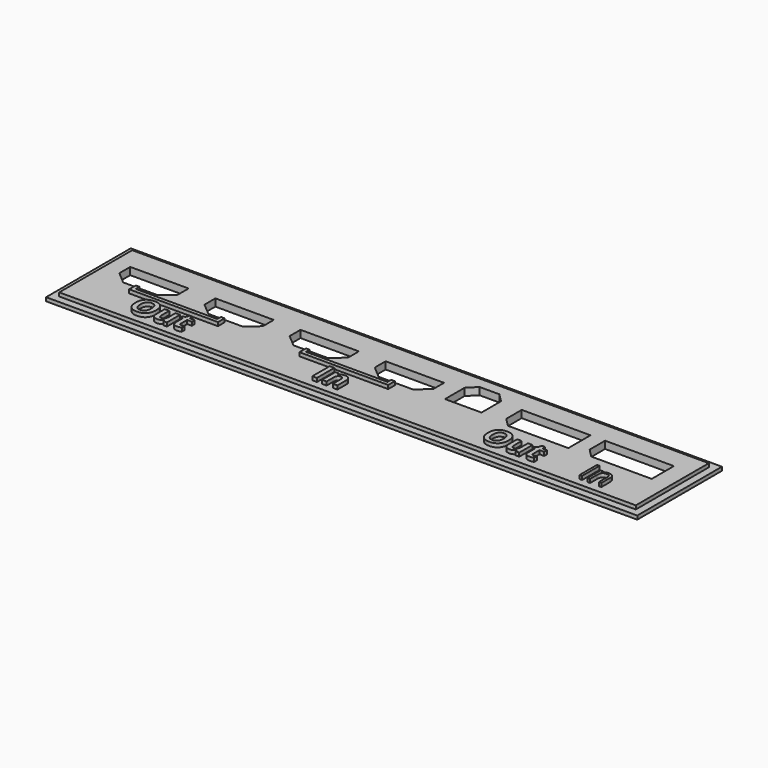
from build123d import *

# Parameters (mm, degrees)
F2_W          = 158
F2_H          = 25
F3_DEPTH      = 2
F2_W_2        = 162
F2_H_2        = 29
F4_DEPTH      = 1
F9_DEPTH      = 2
F10_OFFSET    = 0.5
F11_TEXT_SIZE = 8.3333333333
F12_DEPTH     = 1


# Not quite as in the source:
# - Text() gives the source's letters only with a copy of the font that has no kerning and outlines rounded to 1/6400 em; it was checked with that copy


with BuildPart() as f3:
    # F2 (on Top) → F3 (new body)
    with BuildSketch(Plane.XY):
        with Locations((-79, 12.5)):
            Rectangle(F2_W, F2_H)
    extrude(amount=F3_DEPTH)

    # F2 (on Top) → F4 (join)
    with BuildSketch(Plane.XY):
        with Locations((-79, 12.5)):
            Rectangle(F2_W_2, F2_H_2)
        with Locations((-79, 12.5)):
            Rectangle(F2_W, F2_H, mode=Mode.SUBTRACT)
    extrude(amount=F4_DEPTH)


with BuildPart() as f9:
    # F6 (on face) → F9 (new body, through all)
    with BuildSketch(Plane.XY.offset(2)):
        Polygon((-138, 18.2), (-145.5, 18.2), (-153, 18.2), (-153, 15.2), (-150, 12.65), (-145.5, 12.65), (-141, 12.65), (-138, 15.2), align=None)
    extrude(amount=-F9_DEPTH)


with BuildPart() as f9b:
    # F6 (on face) → F9, piece 2 (new body, through all)
    with BuildSketch(Plane.XY.offset(2)):
        Polygon((-114.67, 18.2), (-122.17, 18.2), (-129.67, 18.2), (-129.67, 15.2), (-126.67, 12.65), (-122.17, 12.65), (-117.67, 12.65), (-114.67, 15.2), align=None)
    extrude(amount=-F9_DEPTH)


with BuildPart() as f9c:
    # F6 (on face) → F9, piece 3 (new body, through all)
    with BuildSketch(Plane.XY.offset(2)):
        Polygon((-91.34, 18.2), (-98.84, 18.2), (-106.34, 18.2), (-106.34, 15.2), (-103.34, 12.65), (-98.84, 12.65), (-94.34, 12.65), (-91.34, 15.2), align=None)
    extrude(amount=-F9_DEPTH)


with BuildPart() as f9d:
    # F6 (on face) → F9, piece 4 (new body, through all)
    with BuildSketch(Plane.XY.offset(2)):
        Polygon((-68.01, 18.2), (-75.51, 18.2), (-83.01, 18.2), (-83.01, 15.2), (-80.01, 12.65), (-75.51, 12.65), (-71.01, 12.65), (-68.01, 15.2), align=None)
    extrude(amount=-F9_DEPTH)


with BuildPart() as f9e:
    # F7 (on face) → F9, piece 5 (new body, through all)
    with BuildSketch(Plane.XY.offset(2)):
        Polygon((-62.15, 13.45), (-57.65, 13.45), (-53.15, 13.45), (-53.15, 19.45), (-55.15, 21.45), (-57.65, 21.45), (-60.15, 21.45), (-62.15, 19.45), align=None)
    extrude(amount=-F9_DEPTH)


with BuildPart() as f9f:
    # F8 (on face) → F9, piece 6 (new body, through all)
    with BuildSketch(Plane.XY.offset(2)):
        Polygon((-5.5, 12.2), (-5.5, 18.8), (-23.35, 18.8), (-23.35, 14.2), (-21.35, 12.2), align=None)
    extrude(amount=-F9_DEPTH)


with BuildPart() as f9g:
    # F8 (on face) → F9, piece 7 (new body, through all)
    with BuildSketch(Plane.XY.offset(2)):
        Polygon((-28.35, 12.2), (-28.35, 18.8), (-46.2, 18.8), (-46.2, 14.2), (-44.2, 12.2), align=None)
    extrude(amount=-F9_DEPTH)


with BuildPart() as f3_1:
    add(f3.part)

    # F10: cut F9, F9b, F9c, F9d, F9g, F9e, F9f, each made larger all round first
    f10_tool = offset(f9.part, amount=F10_OFFSET, kind=Kind.INTERSECTION, mode=Mode.PRIVATE)
    add(f10_tool, mode=Mode.SUBTRACT)
    f10_tool1 = offset(f9b.part, amount=F10_OFFSET, kind=Kind.INTERSECTION, mode=Mode.PRIVATE)
    add(f10_tool1, mode=Mode.SUBTRACT)
    f10_tool2 = offset(f9c.part, amount=F10_OFFSET, kind=Kind.INTERSECTION, mode=Mode.PRIVATE)
    add(f10_tool2, mode=Mode.SUBTRACT)
    f10_tool3 = offset(f9d.part, amount=F10_OFFSET, kind=Kind.INTERSECTION, mode=Mode.PRIVATE)
    add(f10_tool3, mode=Mode.SUBTRACT)
    f10_tool4 = offset(f9g.part, amount=F10_OFFSET, kind=Kind.INTERSECTION, mode=Mode.PRIVATE)
    add(f10_tool4, mode=Mode.SUBTRACT)
    f10_tool5 = offset(f9e.part, amount=F10_OFFSET, kind=Kind.INTERSECTION, mode=Mode.PRIVATE)
    add(f10_tool5, mode=Mode.SUBTRACT)
    f10_tool6 = offset(f9f.part, amount=F10_OFFSET, kind=Kind.INTERSECTION, mode=Mode.PRIVATE)
    add(f10_tool6, mode=Mode.SUBTRACT)

    # F11 (on face) → F12 (join)
    with BuildSketch(Plane.XY.offset(2)):
        Polygon((-146, 11.2277884036), (-146, 8.9637285247), (-133.835, 8.9637285247), (-121.67, 8.9637285247), (-121.67, 11.2277884036), (-122.67, 11.2277884036), (-122.67, 9.9637285247), (-133.835, 9.9637285247), (-145, 9.9637285247), (-145, 11.2277884036), align=None)
        Polygon((-75.01, 11.2277884036), (-76.01, 11.2277884036), (-76.01, 9.9637285247), (-87.175, 9.9637285247), (-98.34, 9.9637285247), (-98.34, 11.2277884036), (-99.34, 11.2277884036), (-99.34, 8.9637285247), (-87.175, 8.9637285247), (-75.01, 8.9637285247), align=None)
        with Locations((-90.9796875, 2)):
            Text('In', F11_TEXT_SIZE, font='Open Sans', font_style=FontStyle.BOLD, text_align=(TextAlign.LEFT, TextAlign.BOTTOM))
        with Locations((-141.5641666667, 2)):
            Text('Out', F11_TEXT_SIZE, font='Open Sans', font_style=FontStyle.BOLD, text_align=(TextAlign.LEFT, TextAlign.BOTTOM))
        with Locations((-45.0041666667, 2)):
            Text('Out', F11_TEXT_SIZE, font='Open Sans', font_style=FontStyle.BOLD, text_align=(TextAlign.LEFT, TextAlign.BOTTOM))
        with Locations((-17.8084635417, 2)):
            Text('In', F11_TEXT_SIZE, font='Open Sans', text_align=(TextAlign.LEFT, TextAlign.BOTTOM))
    extrude(amount=F12_DEPTH)


solid = f3_1.part
